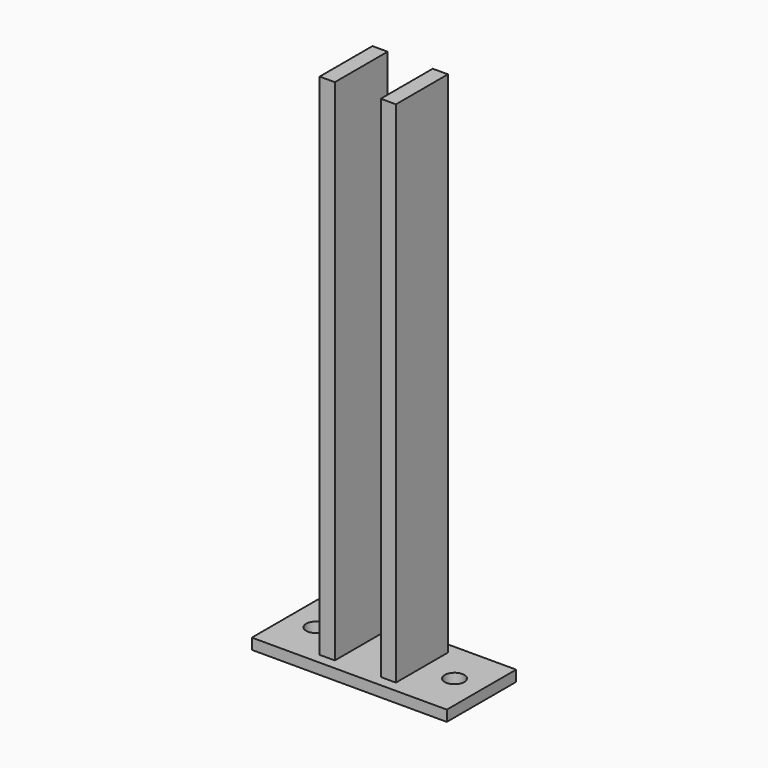
from build123d import *

# Parameters (mm, degrees)
F0_W     = 40
F0_H     = 5
F1_DEPTH = 90
F2_W     = 7
F2_H     = 30.4702166427
F2_H_2   = 30
F3_DEPTH = 240
F5_D     = 9


# Not quite as in the source:
# - a feature names something its author has since deleted; it is built from what else it names


with BuildPart() as f1:
    # F0 (on Right) → F1 (new body)
    with BuildSketch(Plane.YZ):
        with Locations((-0.72813743, 2.5)):
            Rectangle(F0_W, F0_H)
    extrude(amount=F1_DEPTH)

    # F2 (on Top) → F3 (join)
    with BuildSketch(Plane.XY):
        with Locations((31, -0.7447636027)):
            Rectangle(F2_W, F2_H)
        with Locations((59, -0.72813743)):
            Rectangle(F2_W, F2_H_2)
    extrude(amount=F3_DEPTH)

    # F5 (through all)
    with Locations(Plane(origin=(0, 0, 0), x_dir=(1, 0, 0), z_dir=(0, 0, -1))):
        with Locations((13, 0), (77, 0)):
            Hole(F5_D / 2)


solid = f1.part
